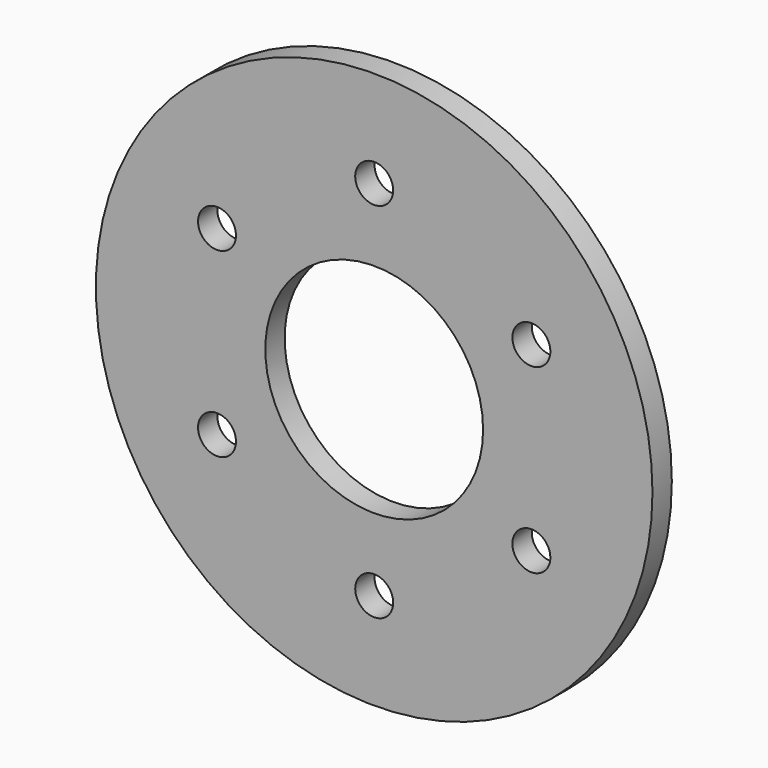
from build123d import *

# Parameters (mm, degrees)
F0_R            = 36.5125
F0_R_2          = 14.2875
F1_DEPTH        = 3.175
F2_R            = 2.4892
F3_DEPTH        = 3.176
F3_COPIES_COUNT = 6


# Not quite as in the source:
# - a pattern or mirror of a feature is missing from the dataset's text; its kind, count and spacing are read off the source's solid


with BuildPart() as f1:
    # F0 (on Front) → F1 (new body)
    with BuildSketch(Plane.XZ):
        Circle(F0_R)
        Circle(F0_R_2, mode=Mode.SUBTRACT)
    extrude(amount=F1_DEPTH)

    # F2 (on face) → F3 (cut, through all)
    with BuildSketch(Plane.XZ.offset(3.175)):
        with Locations((0, 23.8125)):
            Circle(F2_R)
    f3 = extrude(amount=-F3_DEPTH, mode=Mode.SUBTRACT)

    # F3_copies: F3 ×6 about axis
    f3_copies_axis = Axis((0, 0, 0), (0, 1, 0))
    for i in range(1, F3_COPIES_COUNT):
        add(f3.rotate(f3_copies_axis, i * 360 / F3_COPIES_COUNT), mode=Mode.SUBTRACT)


solid = f1.part
